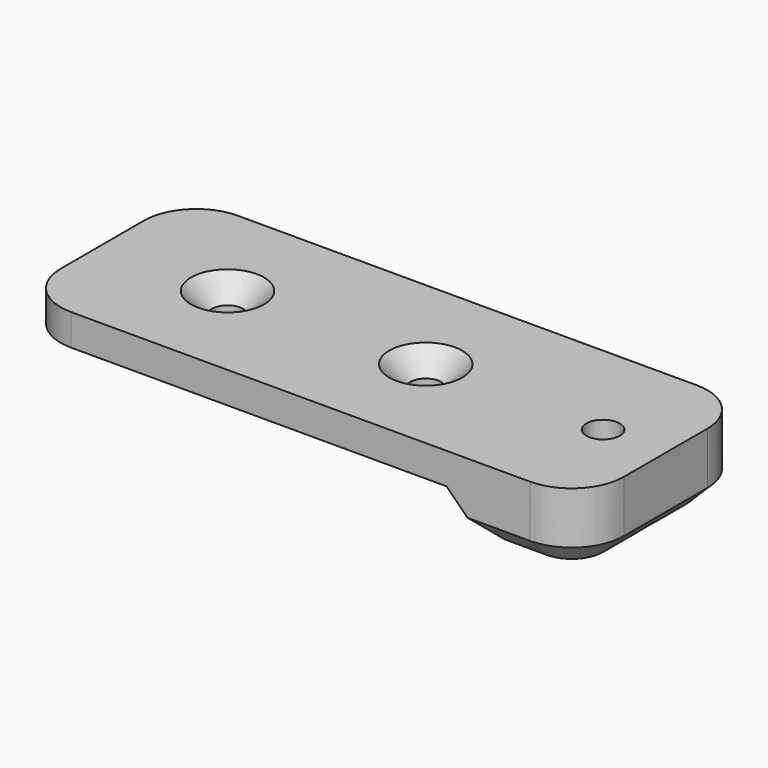
from build123d import *

# Parameters (mm, degrees)
F0_R        = 1.5
F0_R_2      = 1.6
F1_DEPTH    = 3
F2_SIZE     = 2
F3_R        = 4.1
F4_DEPTH    = 4
F5_T4_DEPTH = 40.5734639037
F6_T1_DEPTH = 9.1433659759
F6_T3_DEPTH = 10
F6_T6_ANGLE = 90
F6_T8_ANGLE = 90


# Not quite as in the source:
# - a fillet or chamfer that OpenCascade refuses, or shapes differently, is made with other operations: its cross-section is extruded or revolved along the edge and cut away or added


with BuildPart() as f1:
    # F0 (on Top) → F1 (new body)
    with BuildSketch(Plane.XY):
        with BuildLine():
            Line((22, 10), (-22, 10))
            ThreePointArc((-22, 10), (-25.5355339059, 8.5355339059), (-27, 5))
            Line((-27, 5), (-27, -5))
            ThreePointArc((-27, -5), (-25.5355339059, -8.5355339059), (-22, -10))
            Line((-22, -10), (22, -10))
            ThreePointArc((22, -10), (25.5355339059, -8.5355339059), (27, -5))
            Line((27, -5), (27, 5))
            ThreePointArc((27, 5), (25.5355339059, 8.5355339059), (22, 10))
        make_face()
        with Locations((-15, 0)):
            Circle(F0_R, mode=Mode.SUBTRACT)
        with Locations((4, 0)):
            Circle(F0_R, mode=Mode.SUBTRACT)
        with Locations((21, 0)):
            Circle(F0_R_2, mode=Mode.SUBTRACT)
    extrude(amount=F1_DEPTH)

    # F2
    f2_edges = [f1.edges().sort_by_distance(p)[0] for p in [
        (-16.5, 0, 3),
        (2.5, 0, 3),
    ]]
    chamfer(f2_edges, length=F2_SIZE)

    # F3 (on face) → F4 (join)
    with BuildSketch(Plane(origin=(0, 0, 0), x_dir=(1, 0, 0), z_dir=(0, 0, -1))):
        with BuildLine():
            Line((14, 10), (14, -10))
            Line((14, -10), (22, -10))
            ThreePointArc((22, -10), (25.5355339059, -8.5355339059), (27, -5))
            Line((27, -5), (27, 5))
            ThreePointArc((27, 5), (25.5355339059, 8.5355339059), (22, 10))
            Line((22, 10), (14, 10))
        make_face()
        with Locations((21, 0)):
            Circle(F3_R, mode=Mode.SUBTRACT)
    extrude(amount=F4_DEPTH)

    # F5: chamfer of 4 on 1 edges, made by hand


with BuildPart() as f5_tool2:
    # F5_s3 → F5_t4 (new body)
    with BuildSketch(Plane.XZ.offset(20.2867319519)):
        Polygon((18, -4), (14, 0), (14, -4), align=None)
    extrude(amount=-F5_T4_DEPTH)

    split(bisect_by=Plane.XY, keep=Keep.BOTTOM)


with BuildPart() as f1_1:
    add(f1.part)

    # F5_t1: cut F5_tool2
    add(f5_tool2.part, mode=Mode.SUBTRACT)

    # F6: chamfer of 2 on 5 edges, made by hand

    # F6_s2 → F6_t1 (cut)
    with BuildSketch(Plane.YZ.offset(12.8566340241)):
        Polygon((-10, -2), (-8, -4), (-10, -4), align=None)
        Polygon((10, -2), (8, -4), (10, -4), align=None)
    extrude(amount=F6_T1_DEPTH, mode=Mode.SUBTRACT)

    # F6_s4 → F6_t3 (cut)
    with BuildSketch(Plane.XZ.offset(-5)):
        Polygon((27, -2), (25, -4), (27, -4), align=None)
    extrude(amount=F6_T3_DEPTH, mode=Mode.SUBTRACT)

    # F6_s5 → F6_t6 (revolve, cut)
    with BuildSketch(Plane.XZ.offset(5)):
        Polygon((27, -2), (25, -4), (27, -4), align=None)
    revolve(axis=Axis((22, -5, -4), (0, 0, -1)), revolution_arc=F6_T6_ANGLE, mode=Mode.SUBTRACT)

    # F6_s7 → F6_t8 (revolve, cut)
    with BuildSketch(Plane.YZ.offset(22)):
        Polygon((10, -2), (8, -4), (10, -4), align=None)
    revolve(axis=Axis((22, 5, -4), (0, 0, -1)), revolution_arc=F6_T8_ANGLE, mode=Mode.SUBTRACT)


solid = f1_1.part
